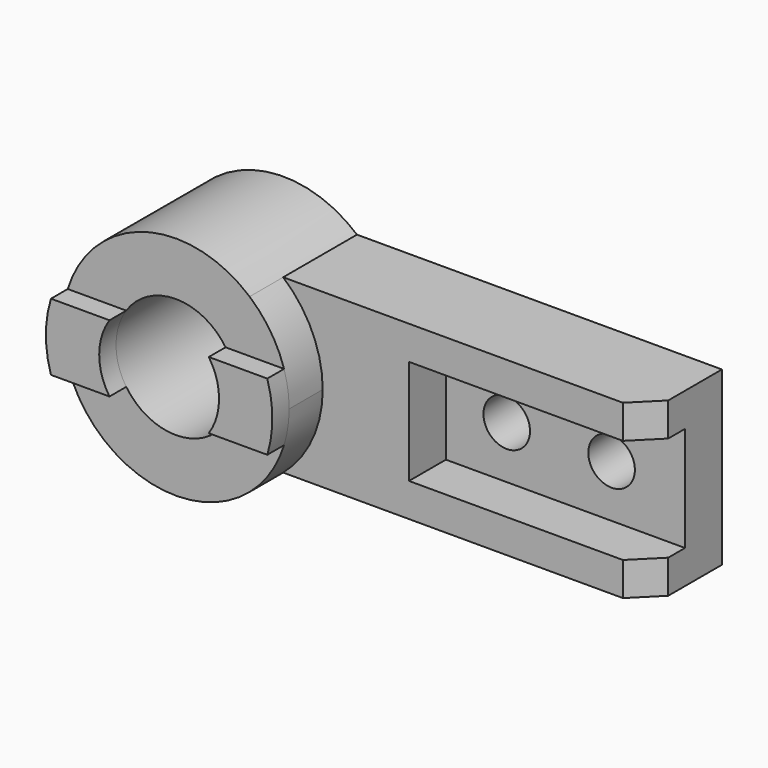
from build123d import *
from build123d import SkipClean  # not in build123d's __all__

# Parameters (mm, degrees)
F0_R          = 28.575
F1_DEPTH      = 64
F2_DEPTH      = 44
F4_W          = 114
F4_H          = 50
F5_DEPTH      = 22
F6_DEPTH      = 95.001
F6_DEPTH_BACK = 25
F7_R          = 11.1
F8_DEPTH      = 22.001
F10_DEPTH     = 10
F12_DEPTH     = 10


# Not quite as in the source:
# - after a boolean that leaves OpenCascade's solid faulty, fix() repairs it


with BuildPart() as f1:
    # F0 (on Front) → F1 (new body)
    with BuildSketch(Plane.XZ):
        with BuildLine():
            ThreePointArc((35.1425667816, -41), (49.0596504584, -22.5643678594), (54, 0))
            ThreePointArc((54, 0), (49.0596504584, 22.5643678594), (35.1425667816, 41))
            ThreePointArc((35.1425667816, 41), (-54, 0), (35.1425667816, -41))
        make_face()
        Circle(F0_R, mode=Mode.SUBTRACT)
    extrude(amount=F1_DEPTH)

    # F0 (on Front) → F2 (join)
    with BuildSketch(Plane.XZ):
        with BuildLine():
            ThreePointArc((35.1425667816, 41), (49.0596504584, 22.5643678594), (54, 0))
            ThreePointArc((54, 0), (49.0596504584, -22.5643678594), (35.1425667816, -41))
            Line((35.1425667816, -41), (209.1425667816, -41))
            Line((209.1425667816, -41), (209.1425667816, 41))
            Line((209.1425667816, 41), (35.1425667816, 41))
        make_face()
    extrude(amount=F2_DEPTH)

    # F4 (on face) → F5 (cut)
    with BuildSketch(Plane.XZ.offset(44)):
        with Locations((152.1425667816, 0)):
            Rectangle(F4_W, F4_H)
    extrude(amount=-F5_DEPTH, mode=Mode.SUBTRACT)

    # F3 (on face) → F6 (cut, two sides)
    with BuildSketch(Plane.XY.offset(41)) as f6_sk:
        Polygon((209.1425667816, -32), (197.1425667816, -44), (209.1425667816, -44), align=None)
    extrude(amount=-F6_DEPTH, mode=Mode.SUBTRACT)
    extrude(f6_sk.sketch, amount=F6_DEPTH_BACK, mode=Mode.SUBTRACT)

    # F7 (on face) → F8 (cut, through all)
    with BuildSketch(Plane.XZ.offset(22)):
        with Locations((124.1425667816, 0)):
            Circle(F7_R)
        with Locations((174.1425667816, 0)):
            Circle(F7_R)
    extrude(amount=-F8_DEPTH, mode=Mode.SUBTRACT)

    # F9 (on face) → F10 (join)
    with BuildSketch(Plane.XZ.offset(64)):
        with BuildLine():
            ThreePointArc((-23.6755279772, -16), (-28.575, 0), (-23.6755279772, 16))
            Line((-23.6755279772, 16), (-51.5751878329, 16))
            ThreePointArc((-51.5751878329, 16), (-54, 0), (-51.5751878329, -16))
            Line((-51.5751878329, -16), (-23.6755279772, -16))
        make_face()
    extrude(amount=F10_DEPTH)

    add(f1.part.fix(), mode=Mode.REPLACE)

    # F11 (on face) → F12 (join)
    with BuildSketch(Plane.XZ.offset(64)):
        with BuildLine():
            ThreePointArc((23.6755279772, 16), (28.575, 0), (23.6755279772, -16))
            Line((23.6755279772, -16), (51.5751878329, -16))
            ThreePointArc((51.5751878329, -16), (54, 0), (51.5751878329, 16))
            Line((51.5751878329, 16), (23.6755279772, 16))
        make_face()
    with SkipClean():  # cleaning this boolean's faces spoils the solid; the shape is the same uncleaned
        extrude(amount=F12_DEPTH)


solid = f1.part
